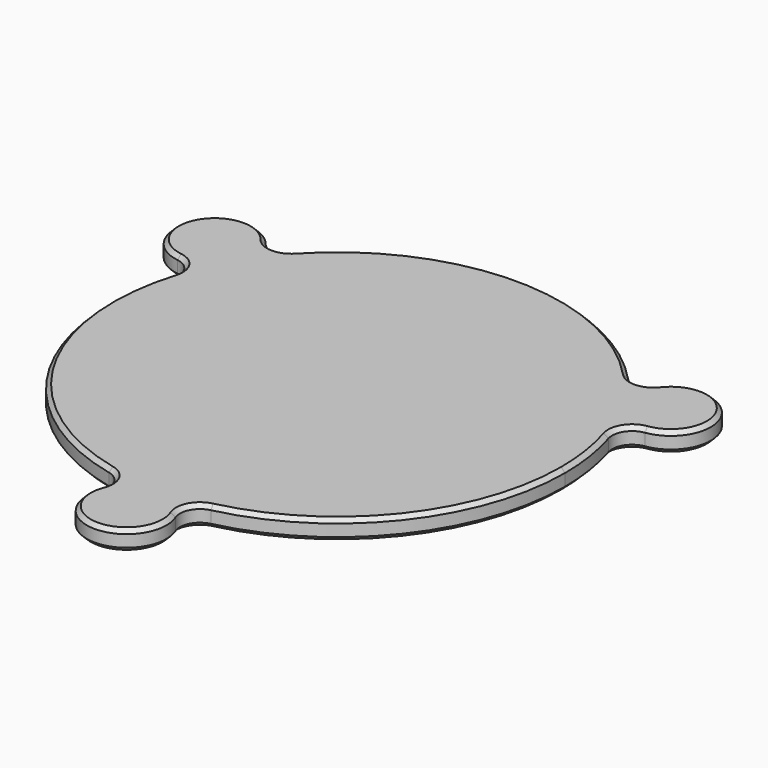
from build123d import *

# Parameters (mm, degrees)
F1_DEPTH = 5
F2_R     = 5
F3_SIZE  = 1


with BuildPart() as f1:
    # F0 (on Top) → F1 (new body)
    with BuildSketch(Plane.XY):
        with BuildLine():
            ThreePointArc((47.3444830059, 32.0097239742), (49.4933518263, 28.575), (51.3934756327, 24.996663025))
            ThreePointArc((51.3934756327, 24.996663025), (65.9478344982, 38.075), (47.3444830059, 32.0097239742))
        make_face()
        with BuildLine():
            ThreePointArc((4.0489926269, -57.0063869992), (41.8181923846, -38.9533218826), (57.15, 0))
            ThreePointArc((57.15, 0), (55.6922778867, 12.8254701198), (51.3934756327, 24.996663025))
            ThreePointArc((51.3934756327, 24.996663025), (49.4933518263, 28.575), (47.3444830059, 32.0097239742))
            ThreePointArc((47.3444830059, 32.0097239742), (0, 57.15), (-47.3444830059, 32.0097239742))
            ThreePointArc((-47.3444830059, 32.0097239742), (-49.4933518263, 28.575), (-51.3934756327, 24.996663025))
            ThreePointArc((-51.3934756327, 24.996663025), (-49.4933518263, -28.575), (-4.0489926269, -57.0063869992))
            ThreePointArc((-4.0489926269, -57.0063869992), (0, -57.15), (4.0489926269, -57.0063869992))
        make_face()
        with BuildLine():
            ThreePointArc((-51.3934756327, 24.996663025), (-49.4933518263, 28.575), (-47.3444830059, 32.0097239742))
            ThreePointArc((-47.3444830059, 32.0097239742), (-65.9478344982, 38.075), (-51.3934756327, 24.996663025))
        make_face()
        with BuildLine():
            ThreePointArc((-4.0489926269, -57.0063869992), (0, -76.15), (4.0489926269, -57.0063869992))
            ThreePointArc((4.0489926269, -57.0063869992), (0, -57.15), (-4.0489926269, -57.0063869992))
        make_face()
    extrude(amount=F1_DEPTH)

    # F2
    f2_edges = [f1.edges().sort_by_distance(p)[0] for p in [
        (-4.048993, -57.006387, 2.5),
        (-47.344483, 32.009724, 2.5),
        (51.393476, 24.996663, 2.5),
        (47.344483, 32.009724, 2.5),
        (-51.393476, 24.996663, 2.5),
        (4.048993, -57.006387, 2.5),
    ]]
    fillet(f2_edges, radius=F2_R)

    # F3
    f3_edges = [f1.edges().sort_by_distance(p)[0] for p in [
        (65.947834, 38.075, 5),
        (55.195163, 20.905484, 5),
        (45.702262, 37.347671, 5),
        (49.493352, -28.575, 5),
        (0, 57.15, 5),
        (9.492901, -58.253155, 5),
        (-45.702262, 37.347671, 5),
        (0, -76.15, 5),
        (-65.947834, 38.075, 5),
        (-9.492901, -58.253155, 5),
        (-55.195163, 20.905484, 5),
        (-49.493352, -28.575, 5),
        (65.947834, 38.075, 0),
        (55.195163, 20.905484, 0),
        (45.702262, 37.347671, 0),
        (49.493352, -28.575, 0),
        (0, 57.15, 0),
        (9.492901, -58.253155, 0),
        (-45.702262, 37.347671, 0),
        (0, -76.15, 0),
        (-65.947834, 38.075, 0),
        (-9.492901, -58.253155, 0),
        (-55.195163, 20.905484, 0),
        (-49.493352, -28.575, 0),
    ]]
    chamfer(f3_edges, length=F3_SIZE)


solid = f1.part
